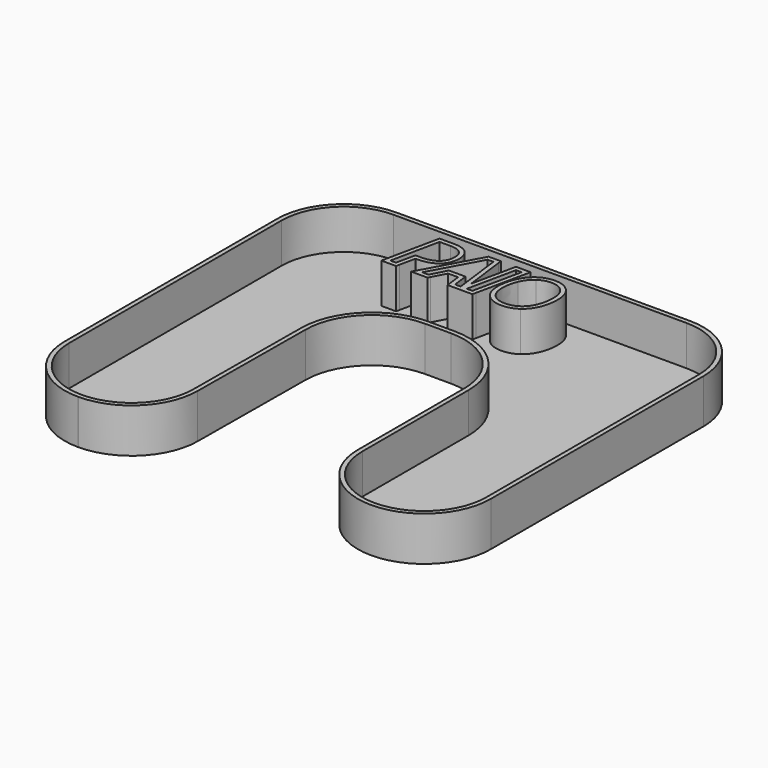
from build123d import *

# Parameters (mm, degrees)
F1_DEPTH    = 10
F2_T        = 1
F2_T3_DEPTH = 12


# Not quite as in the source:
# - a shell that OpenCascade refuses in one call is made with other operations: the cavity is built on its own and cut out


with BuildPart() as f1:
    # F0 (on Top) → F1 (new body)
    with BuildSketch(Plane.XY):
        with BuildLine():
            ThreePointArc((0, 15), (4.3933982822, 4.3933982822), (15, 0))
            Line((15, 0), (15.1102871592, 0))
            ThreePointArc((15.1102871592, 0), (25.6776806682, 4.3543344771), (30.1098787254, 14.8893074099))
            Line((30.1098787254, 14.8893074099), (30.3329036916, 45.1106925901))
            ThreePointArc((30.3329036916, 45.1106925901), (34.7651017487, 55.6456655229), (45.3324952577, 60))
            Line((45.3324952577, 60), (51.1982429028, 60))
            ThreePointArc((51.1982429028, 60), (61.8048446206, 55.6066017178), (66.1982429028, 45))
            Line((66.1982429028, 45), (66.1982429028, 15))
            ThreePointArc((66.1982429028, 15), (70.591641185, 4.3933982822), (81.1982429028, 0))
            ThreePointArc((81.1982429028, 0), (91.8048446206, 4.3933982822), (96.1982429028, 15))
            Line((96.1982429028, 15), (96.1982429028, 75))
            ThreePointArc((96.1982429028, 75), (91.8048446206, 85.6066017178), (81.1982429028, 90))
            Line((81.1982429028, 90), (15, 90))
            ThreePointArc((15, 90), (4.3933982822, 85.6066017178), (0, 75))
            Line((0, 75), (0, 15))
        make_face()
        with BuildLine():
            add(Edge.make_bspline(
                [(32.7684162624, 85.269208592), (33.5950473039, 84.5591229154), (33.5950473039, 83.148563551)],
                knots=[0, 0, 0, 1, 1, 1], degree=2))
            add(Edge.make_bspline(
                [(33.5950473039, 83.148563551), (33.5950473039, 81.2862407106), (32.363511232, 80.3022133516)],
                knots=[0, 0, 0, 1, 1, 1], degree=2))
            add(Edge.make_bspline(
                [(32.363511232, 80.3022133516), (31.13197516, 79.3181859927), (28.7506049214, 79.3181859927)],
                knots=[0, 0, 0, 1, 1, 1], degree=2))
            Line((28.7506049214, 79.3181859927), (27.7365400973, 79.3181859927))
            Line((27.7365400973, 79.3181859927), (26.8137891673, 75))
            Line((26.8137891673, 75), (25.537797647, 75))
            Line((25.537797647, 75), (27.856689958, 85.9792942686))
            Line((27.856689958, 85.9792942686), (30.3365830824, 85.9792942686))
            add(Edge.make_bspline(
                [(30.3365830824, 85.9792942686), (31.941785221, 85.9792942686), (32.7684162624, 85.269208592)],
                knots=[0, 0, 0, 1, 1, 1], degree=2))
        make_face(mode=Mode.SUBTRACT)
        Polygon((40.1287967274, 75), (39.7010632234, 78.4915549512), (35.9764175425, 78.4915549512), (34.1357216769, 75), (32.7155503237, 75), (38.7158343659, 85.9792942686), (40.0230648501, 85.9792942686), (41.4047882478, 75), align=None, mode=Mode.SUBTRACT)
        Polygon((44.0408761911, 75), (42.779302654, 75), (45.1150159455, 85.9792942686), (46.3765894826, 85.9792942686), align=None, mode=Mode.SUBTRACT)
        with BuildLine():
            add(Edge.make_bspline(
                [(55.874435969, 84.9952669096), (56.9257472499, 83.8382237513), (56.9257472499, 81.8100941031)],
                knots=[0, 0, 0, 1, 1, 1], degree=2))
            add(Edge.make_bspline(
                [(56.9257472499, 81.8100941031), (56.9257472499, 79.7915764438), (56.2649230162, 78.195986294)],
                knots=[0, 0, 0, 1, 1, 1], degree=2))
            add(Edge.make_bspline(
                [(56.2649230162, 78.195986294), (55.6040987825, 76.6003961442), (54.3725627106, 75.7245036599)],
                knots=[0, 0, 0, 1, 1, 1], degree=2))
            add(Edge.make_bspline(
                [(54.3725627106, 75.7245036599), (53.1410266387, 74.8486111755), (51.5286155084, 74.8486111755)],
                knots=[0, 0, 0, 1, 1, 1], degree=2))
            add(Edge.make_bspline(
                [(51.5286155084, 74.8486111755), (49.6062177376, 74.8486111755), (48.5320779831, 75.9720123729)],
                knots=[0, 0, 0, 1, 1, 1], degree=2))
            add(Edge.make_bspline(
                [(48.5320779831, 75.9720123729), (47.4579382287, 77.0954135702), (47.4579382287, 79.1235432184)],
                knots=[0, 0, 0, 1, 1, 1], degree=2))
            add(Edge.make_bspline(
                [(47.4579382287, 79.1235432184), (47.4579382287, 81.1060159196), (48.1788373927, 82.742457022)],
                knots=[0, 0, 0, 1, 1, 1], degree=2))
            add(Edge.make_bspline(
                [(48.1788373927, 82.742457022), (48.8997365568, 84.3788981244), (50.1577055981, 85.2656040962)],
                knots=[0, 0, 0, 1, 1, 1], degree=2))
            add(Edge.make_bspline(
                [(50.1577055981, 85.2656040962), (51.4156746393, 86.1523100679), (52.9920408114, 86.1523100679)],
                knots=[0, 0, 0, 1, 1, 1], degree=2))
            add(Edge.make_bspline(
                [(52.9920408114, 86.1523100679), (54.8231246881, 86.1523100679), (55.874435969, 84.9952669096)],
                knots=[0, 0, 0, 1, 1, 1], degree=2))
        make_face(mode=Mode.SUBTRACT)
    extrude(amount=F1_DEPTH)

    # F2: shell of thickness 1, made by hand


with BuildPart() as f2_core1:
    # F2_t2: copy of F1
    add(f1.part)

    # the walls: a layer under each face that stays
    f2_faces = [f2_core1.faces().sort_by_distance(p)[0] for p in [
        (4.3933982822, 4.3933982822, 5),
        (54.6281815392, 85.8630492784, 5),
        (51.495273922, 85.930633575, 5),
        (49.0340040261, 84.1914643417, 5),
        (47.6381630197, 81.0195080199, 5),
        (47.7264731673, 77.3215956829, 5),
        (49.8182822417, 75.1294614749, 5),
        (53.0458078741, 75.0675842966, 5),
        (55.461420823, 76.7803205606, 5),
        (56.7605411915, 79.8973083212, 5),
        (56.6629194297, 83.6204521288, 5),
        (45.2087328368, 80.4896471343, 5),
        (45.745802714, 85.9792942686, 5),
        (43.9471592997, 80.4896471343, 5),
        (43.4100894225, 75, 5),
        (40.7667924876, 75, 5),
        (40.7139265489, 80.4896471343, 5),
        (39.369449608, 85.9792942686, 5),
        (35.7156923448, 80.4896471343, 5),
        (33.4256360003, 75, 5),
        (35.0560696097, 76.7457774756, 5),
        (37.838740383, 78.4915549512, 5),
        (39.9149299754, 76.7457774756, 5),
        (31.7471424467, 85.8017728494, 5),
        (29.0966365202, 85.9792942686, 5),
        (26.6972438025, 80.4896471343, 5),
        (26.1757934071, 75, 5),
        (27.2751646323, 77.1590929963, 5),
        (28.2435725094, 79.3181859927, 5),
        (30.8445166184, 79.5641928324, 5),
        (33.2871632859, 81.505814581, 5),
        (33.3883895435, 84.3840044934, 5),
        (4.3933982822, 85.6066017178, 5),
        (48.0991214514, 90, 5),
        (91.8048446206, 85.6066017178, 5),
        (96.1982429028, 45, 5),
        (81.1982429028, 0, 5),
        (66.1982429028, 30, 5),
        (61.8048446206, 55.6066017178, 5),
        (48.2653690802, 60, 5),
        (34.7651017487, 55.6456655229, 5),
        (30.2213912085, 30, 5),
        (25.6776806682, 4.3543344771, 5),
        (16.0330404838, 15, 0),
        (15.0551435796, 0, 5),
        (0, 45, 5),
    ]]
    thicken(f2_faces, amount=-F2_T, mode=Mode.SUBTRACT)

    # F2_s4 → F2_t3 (cut)
    with BuildSketch(Plane.XY.offset(-1)):
        Polygon((46.3668083677, 85.9713750836), (47.354700974, 85.7712127694), (47.6117058366, 86.9792942686), (46.3765894826, 86.9792942686), align=None)
        Polygon((44.0310950761, 75.012080815), (45.0189876825, 74.7919185008), (44.850516511, 74), (44.0408761911, 74), align=None)
        Polygon((45.1247970604, 85.9672134536), (45.1150159455, 86.9792942686), (44.3053756256, 86.9792942686), (44.1369044541, 86.1873757677), align=None)
        Polygon((42.7890837689, 75.007919185), (41.8011911625, 75.2080814992), (41.5441862999, 74), (42.779302654, 74), align=None)
        Polygon((41.3948665082, 75.0087513678), (41.4047882478, 74), (42.5385241192, 74), (42.3969622132, 75.1248632152), align=None)
        Polygon((40.138722524, 75.0112159613), (40.1287967274, 74), (39.2438260758, 74), (39.1362170678, 74.8784038683), align=None)
        Polygon((40.0131431104, 85.9680456364), (41.0152388154, 86.1041574837), (40.9051045078, 86.9792942686), (40.0230648501, 86.9792942686), align=None)
        Polygon((38.7246094287, 85.9644986171), (38.7158343659, 86.9792942686), (38.1227504611, 86.9792942686), (37.8383280889, 86.4588594193), align=None)
        Polygon((32.7243253865, 75.0052043485), (31.8380440467, 75.4795651507), (31.029448253, 74), (32.7155503237, 74), align=None)
        Polygon((34.1268756663, 75.0146634853), (34.1357216769, 74), (34.7389896226, 74), (35.0203227434, 74.5336514681), align=None)
        Polygon((27.8664741133, 85.9672277967), (27.856689958, 86.9792942686), (27.0458352698, 86.9792942686), (26.878274432, 86.1859414523), align=None)
        Polygon((25.5475818022, 75.0079335282), (24.559382121, 75.2066471838), (24.3045310524, 74), (25.537797647, 74), align=None)
        Polygon((26.8040099502, 75.0120897158), (26.8137891673, 74), (27.6226764277, 74), (27.7917108803, 74.7910284153), align=None)
    extrude(amount=F2_T3_DEPTH, mode=Mode.SUBTRACT)


with BuildPart() as f1_1:
    add(f1.part)

    # what is left inside the walls is the cavity
    f2_cavity = [f2_core1.part.solids().sort_by_distance(p)[0] for p in [
        (24.549561, 59.666667, 9.99),
    ]]
    add(f2_cavity, mode=Mode.SUBTRACT)


solid = f1_1.part
